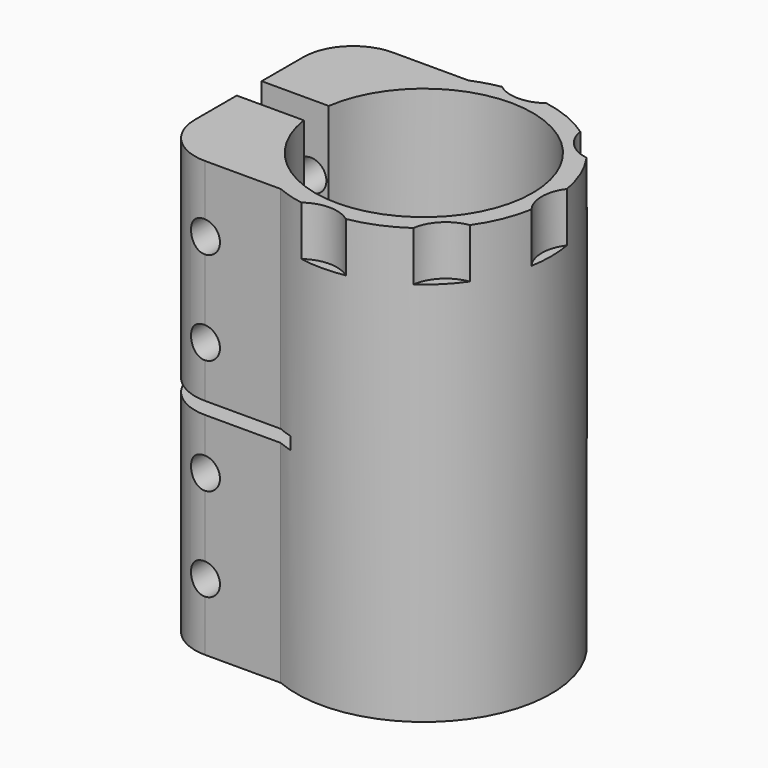
from build123d import *
from build123d import SkipClean  # not in build123d's __all__

# Parameters (mm, degrees)
F1_DEPTH       = 35
F3_D           = 5
F3_START       = 1.8205079
F3_CBORE_D     = 10
F3_CBORE_DEPTH = 8
F4_W           = 22.4
F4_H           = 2
F5_DEPTH       = 25
F6_R           = 6
F7_DEPTH       = 8


with BuildPart() as f1:
    # F0 (on Top) → F1 (new body, symmetric)
    with BuildSketch(Plane.XY):
        with BuildLine():
            Line((-20.1192642082, -18.9086026559), (-7.9192642082, -18.9086026559))
            ThreePointArc((-7.9192642082, -18.9086026559), (20.5, 0), (-7.9192642082, 18.9086026559))
            Line((-7.9192642082, 18.9086026559), (-20.1192642082, 18.9086026559))
            ThreePointArc((-20.1192642082, 18.9086026559), (-25.7761184577, 16.5654569054), (-28.1192642082, 10.9086026559))
            Line((-28.1192642082, 10.9086026559), (-28.1192642082, 2.5086026559))
            Line((-28.1192642082, 2.5086026559), (-17.3192642082, 2.5086026559))
            ThreePointArc((-17.3192642082, 2.5086026559), (1.2575524553, 17.4547575698), (17.5, 0))
            ThreePointArc((17.5, 0), (1.2575524553, -17.4547575698), (-17.3192642082, -2.5086026559))
            Line((-17.3192642082, -2.5086026559), (-28.1192642082, -2.5086026559))
            Line((-28.1192642082, -2.5086026559), (-28.1192642082, -10.9086026559))
            ThreePointArc((-28.1192642082, -10.9086026559), (-25.7761184577, -16.5654569054), (-20.1192642082, -18.9086026559))
        make_face()
    extrude(amount=F1_DEPTH, both=True)

    # F3 (through all)
    # its depths count from where the whole tool has entered the part; down to there all is cleared
    with Locations(Plane(origin=(0, 18.9086026559, 0), x_dir=(-1, 0, 0), z_dir=(0, 1, 0)).offset(-F3_START)):
        with Locations((20.2, -24.25), (20.2, -9.25), (20.2, 9.25), (20.2, 24.25)):
            CounterBoreHole(F3_D / 2, F3_CBORE_D / 2, F3_CBORE_DEPTH)

    # F4 (on Front) → F5 (cut, symmetric)
    with BuildSketch(Plane.XZ):
        with Locations((-16.9192642082, 0)):
            Rectangle(F4_W, F4_H)
    with SkipClean():  # cleaning this boolean's faces spoils the solid; the shape is the same uncleaned
        extrude(amount=F5_DEPTH, both=True, mode=Mode.SUBTRACT)

    # F6 (on face) → F7 (cut)
    with BuildSketch(Plane.XY.offset(35)):
        with Locations((0, -25)):
            Circle(F6_R)
        with Locations((17.6776695297, -17.6776695297)):
            Circle(F6_R)
        with Locations((25, 0)):
            Circle(F6_R)
        with Locations((17.6776695297, 17.6776695297)):
            Circle(F6_R)
        with Locations((0, 25)):
            Circle(F6_R)
    extrude(amount=-F7_DEPTH, mode=Mode.SUBTRACT)


solid = f1.part
